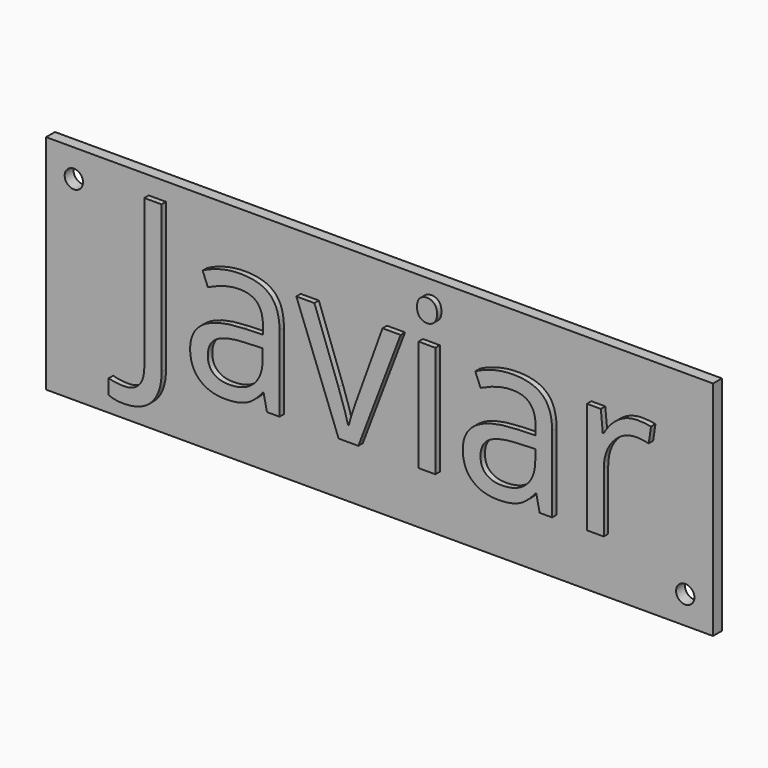
from build123d import *

# Parameters (mm, degrees)
F0_W         = 120
F0_H         = 40
F1_DEPTH     = 2
F3_D         = 3.3
F4_TEXT_SIZE = 37.4509918661
F5_DEPTH     = 1


# Not quite as in the source:
# - Text() gives the source's letters only with a copy of the font that has no kerning and outlines rounded to 1/6400 em; it was checked with that copy


with BuildPart() as f1:
    # F0 (on Front) → F1 (new body)
    with BuildSketch(Plane.XZ):
        Rectangle(F0_W, F0_H)
    extrude(amount=F1_DEPTH)

    # F3 (through all)
    with Locations(Plane.XZ.offset(2)):
        with Locations((-55, 15), (55, -15)):
            Hole(F3_D / 2)

    # F4 (on face) → F5 (join)
    with BuildSketch(Plane.XZ.offset(2)):
        with Locations((-45, -9.9647141436)):
            Text('Javiar', F4_TEXT_SIZE, font='Open Sans', text_align=(TextAlign.LEFT, TextAlign.BOTTOM))
    extrude(amount=F5_DEPTH)


solid = f1.part
